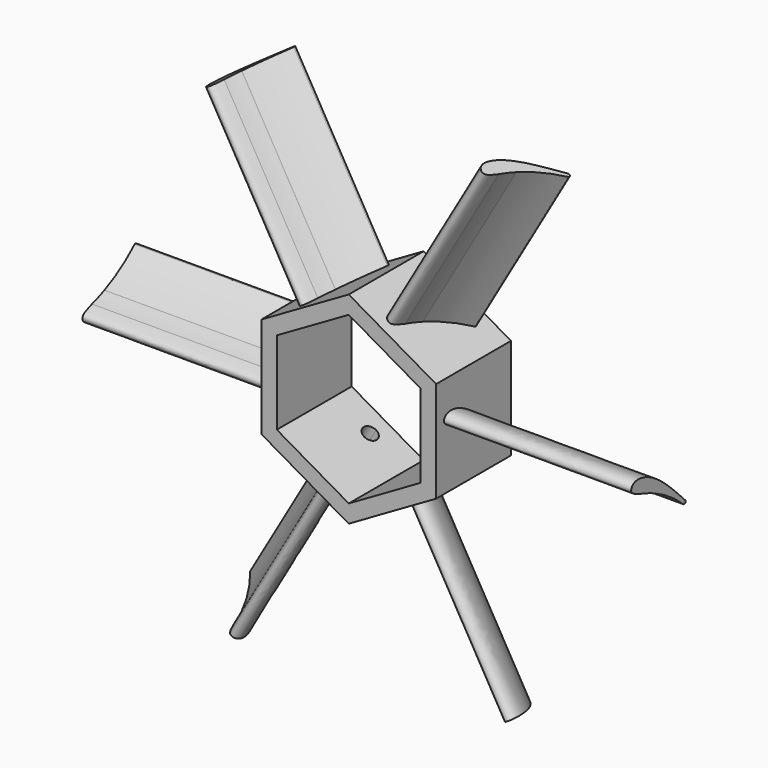
from build123d import *

# Parameters (mm, degrees)
F1_DEPTH  = 19.05
F8_DEPTH  = 38.1
F9_DEPTH  = 38.1
F10_DEPTH = 38.1
F11_DEPTH = 38.1
F12_DEPTH = 38.1
F13_DEPTH = 38.1
F15_DEPTH = 19.0510001
F16_DEPTH = 89.8612751667


# Not quite as in the source:
# - a feature of the source that left no trace in its solid (it failed there, or was rolled back) is left out


with BuildPart() as f1:
    # F0 (on Front) → F1 (new body)
    with BuildSketch(Plane.XZ):
        Polygon((17.78, -10.2652877862), (17.78, 10.2652877862), (0, 20.5305755724), (-17.78, 10.2652877862), (-17.78, -10.2652877862), (0, -20.5305755724), align=None)
    extrude(amount=F1_DEPTH)

    # F7 (on face) → F8 (join)
    with BuildSketch(Plane(origin=(-8.89, 0, 15.3979316793), x_dir=(0.8660254038, 0, 0.5), z_dir=(-0.5, 0, 0.8660254038))):
        with BuildLine():
            add(Edge.make_bspline(
                [(0, -7.7538370491), (0.0005473534, -7.7532338055), (0.0010947416, -7.7526305605), (0.0016421645, -7.7520273142)],
                knots=[0.7876107373, 0.7876107373, 0.7876107373, 0.7876107373, 0.7876968979, 0.7876968979, 0.7876968979, 0.7876968979], degree=3))
            Line((0, -7.7538370491), (0, -11.3412338568))
            ThreePointArc((0, -11.3412338568), (0.0008210147, -11.3393859842), (0.0016421645, -11.3375381715))
            Line((0.0016421645, -11.3375381715), (0.0016421645, -7.7520273142))
        make_face()
        with BuildLine():
            Line((0, -11.3412338568), (0, -7.7538370491))
            add(Edge.make_bspline(
                [(-1.1862251705, -14.5249951817), (-1.5749463751, -15.6161587285), (-2.2464066272, -17.5009876017), (-4.5376219484, -16.1747046), (-3.6264374582, -12.1661122368), (-1.1945785451, -9.0703938169), (0, -7.7538370491)],
                knots=[0, 0, 0, 0, 0.1986769511, 0.3431860009, 0.5995685898, 0.7876107373, 0.7876107373, 0.7876107373, 0.7876107373], degree=3))
            ThreePointArc((-1.1862251705, -14.5249951817), (-0.6420119978, -12.9148952786), (0, -11.3412338568))
        make_face()
        with BuildLine():
            add(Edge.make_bspline(
                [(0.0016421645, -7.7520273142), (1.3505150143, -6.2656031483), (2.9104228785, -4.7706214018), (4.4703307428, -3.2756396553)],
                knots=[0.7876968979, 0.7876968979, 0.7876968979, 0.7876968979, 1, 1, 1, 1], degree=3))
            Line((0.0016421645, -7.7520273142), (0.0016421645, -11.3375381715))
            ThreePointArc((0.0016421645, -11.3375381715), (2.2311378018, -7.2759469782), (5.1069300621, -3.6431804437))
            ThreePointArc((5.1069300621, -3.6431804437), (4.9724007966, -3.1411103898), (4.4703307428, -3.2756396553))
        make_face()
    extrude(amount=F8_DEPTH)

    # F2 (on face) → F9 (join)
    with BuildSketch(Plane(origin=(8.89, 0, 15.3979316793), x_dir=(0.8660254038, 0, -0.5), z_dir=(0.5, 0, 0.8660254038))):
        with BuildLine():
            Line((0, -11.3170660089), (0, -7.7315551515))
            add(Edge.make_bspline(
                [(-1.187867335, -14.5045230191), (-1.5765885396, -15.5956865658), (-2.2480487917, -17.4805154391), (-4.5392641129, -16.1542324374), (-3.6279463171, -12.1450536205), (-1.1952777162, -9.0487213191), (0, -7.7315551515)],
                knots=[0, 0, 0, 0, 0.1986769511, 0.3431860009, 0.5995685898, 0.7876968979, 0.7876968979, 0.7876968979, 0.7876968979], degree=3))
            ThreePointArc((-1.187867335, -14.5045230191), (-0.6429481144, -12.8925283349), (0, -11.3170660089))
        make_face()
        with BuildLine():
            add(Edge.make_bspline(
                [(0, -7.7315551515), (1.3488728498, -6.2451309857), (2.9087807141, -4.7501492392), (4.4686885783, -3.2551674926)],
                knots=[0.7876968979, 0.7876968979, 0.7876968979, 0.7876968979, 1, 1, 1, 1], degree=3))
            Line((0, -7.7315551515), (0, -11.3170660089))
            ThreePointArc((0, -11.3170660089), (2.2294956373, -7.2554748155), (5.1052878976, -3.622708281))
            ThreePointArc((5.1052878976, -3.622708281), (4.9707586321, -3.1206382272), (4.4686885783, -3.2551674926))
        make_face()
    extrude(amount=F9_DEPTH)

    # F3 (on face) → F10 (join)
    with BuildSketch(Plane.YZ.offset(17.78)):
        with BuildLine():
            add(Edge.make_bspline(
                [(-7.8599847579, 0), (-6.3747627763, -1.3481141297), (-4.8810042018, -2.9067457003), (-3.3872456274, -4.4653772708)],
                knots=[0.7878706011, 0.7878706011, 0.7878706011, 0.7878706011, 1, 1, 1, 1], degree=3))
            Line((-7.8599847579, 0), (-11.4416964799, 0))
            ThreePointArc((-11.4416964799, 0), (-7.3841573188, -2.2284377273), (-3.7547864157, -5.1019765901))
            ThreePointArc((-3.7547864157, -5.1019765901), (-3.2527163619, -4.9674473247), (-3.3872456274, -4.4653772708))
        make_face()
        with BuildLine():
            Line((-11.4416964799, 0), (-7.8599847579, 0))
            add(Edge.make_bspline(
                [(-7.8633458805, 0.0030504953), (-7.8622255112, 0.0020337834), (-7.8611051369, 0.0010169516), (-7.8599847579, 0)],
                knots=[0.7877105811, 0.7877105811, 0.7877105811, 0.7877105811, 0.7878706011, 0.7878706011, 0.7878706011, 0.7878706011], degree=3))
            Line((-7.8633458805, 0.0030504953), (-11.4485573206, 0.0030504953))
            ThreePointArc((-11.4485573206, 0.0030504953), (-11.4451267968, 0.0015254803), (-11.4416964799, 0))
        make_face()
        with BuildLine():
            Line((-11.4485573206, 0.0030504953), (-7.8633458805, 0.0030504953))
            add(Edge.make_bspline(
                [(-14.6366011538, 1.1911786424), (-15.7277647005, 1.5798998471), (-17.6125935738, 2.2513600991), (-16.2863105721, 4.5425754204), (-12.2770386202, 3.6312364543), (-9.1806088275, 1.1984392543), (-7.8633458805, 0.0030504953)],
                knots=[0, 0, 0, 0, 0.1986769511, 0.3431860009, 0.5995685898, 0.7877105811, 0.7877105811, 0.7877105811, 0.7877105811], degree=3))
            ThreePointArc((-14.6366011538, 1.1911786424), (-13.0243055984, 0.6461472944), (-11.4485573206, 0.0030504953))
        make_face()
    extrude(amount=F10_DEPTH)

    # F4 (on face) → F11 (join)
    with BuildSketch(Plane(origin=(8.89, 0, -15.3979316793), x_dir=(0.8660254038, 0, 0.5), z_dir=(0.5, 0, -0.8660254038))):
        with BuildLine():
            add(Edge.make_bspline(
                [(0, 7.7183126767), (-1.3479724171, 6.2333150924), (-2.9063657613, 4.7397848289), (-4.4647591055, 3.2462545654)],
                knots=[0.7879030237, 0.7879030237, 0.7879030237, 0.7879030237, 1, 1, 1, 1], degree=3))
            Line((0, 7.7183126767), (0, 11.2993157186))
            ThreePointArc((0, 11.2993157186), (-2.2282401234, 7.2425326354), (-5.1013584248, 3.6137953538))
            ThreePointArc((-5.1013584248, 3.6137953538), (-4.9668291593, 3.1117253), (-4.4647591055, 3.2462545654))
        make_face()
        with BuildLine():
            Line((0, 11.2993157186), (0, 7.7183126767))
            add(Edge.make_bspline(
                [(0.0039294728, 7.7226422243), (0.0026198474, 7.7211990498), (0.0013100231, 7.7197558673), (0, 7.7183126767)],
                knots=[0.7876968979, 0.7876968979, 0.7876968979, 0.7876968979, 0.7879030237, 0.7879030237, 0.7879030237, 0.7879030237], degree=3))
            Line((0.0039294728, 7.7226422243), (0.0039294728, 11.3081530816))
            ThreePointArc((0.0039294728, 11.3081530816), (0.0019651224, 11.3037342285), (0, 11.2993157186))
        make_face()
        with BuildLine():
            Line((0.0039294728, 11.3081530816), (0.0039294728, 7.7226422243))
            add(Edge.make_bspline(
                [(1.1917968078, 14.4956100919), (1.5805180124, 15.5867736386), (2.2519782645, 17.4716025119), (4.5431935857, 16.1453195102), (3.63187579, 12.1361406932), (1.199207189, 9.0398083919), (0.0039294728, 7.7226422243)],
                knots=[0, 0, 0, 0, 0.1986769511, 0.3431860009, 0.5995685898, 0.7876968979, 0.7876968979, 0.7876968979, 0.7876968979], degree=3))
            ThreePointArc((1.1917968078, 14.4956100919), (0.6468775872, 12.8836154077), (0.0039294728, 11.3081530816))
        make_face()
    extrude(amount=F11_DEPTH)

    # F5 (on face) → F12 (join)
    with BuildSketch(Plane(origin=(-8.89, 0, -15.3979316793), x_dir=(0.8660254038, 0, -0.5), z_dir=(-0.5, 0, -0.8660254038))):
        with BuildLine():
            add(Edge.make_bspline(
                [(0, 7.7773641781), (-0.0019872196, 7.7751733378), (-0.0039748984, 7.7729824789), (-0.0059630356, 7.7707916014)],
                knots=[0.787383979, 0.787383979, 0.787383979, 0.787383979, 0.7876968979, 0.7876968979, 0.7876968979, 0.7876968979], degree=3))
            Line((0, 7.7773641781), (0, 11.3697292081))
            ThreePointArc((0, 11.3697292081), (-0.0029806269, 11.3630154378), (-0.0059630356, 11.3563024588))
            Line((-0.0059630356, 11.3563024588), (-0.0059630356, 7.7707916014))
        make_face()
        with BuildLine():
            Line((0, 11.3697292081), (0, 7.7773641781))
            add(Edge.make_bspline(
                [(1.1819042994, 14.543759469), (1.570625504, 15.6349230157), (2.2420857561, 17.519751889), (4.5333010773, 16.1934688873), (3.6224674222, 12.18641996), (1.1927388288, 9.092317135), (0, 7.7773641781)],
                knots=[0, 0, 0, 0, 0.1986769511, 0.3431860009, 0.5995685898, 0.787383979, 0.787383979, 0.787383979, 0.787383979], degree=3))
            ThreePointArc((1.1819042994, 14.543759469), (0.6395493316, 12.9386483491), (0, 11.3697292081))
        make_face()
        with BuildLine():
            add(Edge.make_bspline(
                [(-0.0059630356, 7.7707916014), (-1.3548358854, 6.2843674356), (-2.9147437496, 4.7893856891), (-4.4746516139, 3.2944039425)],
                knots=[0.7876968979, 0.7876968979, 0.7876968979, 0.7876968979, 1, 1, 1, 1], degree=3))
            Line((-0.0059630356, 7.7707916014), (-0.0059630356, 11.3563024588))
            ThreePointArc((-0.0059630356, 11.3563024588), (-2.2354586728, 7.2947112654), (-5.1112509332, 3.6619447309))
            ThreePointArc((-5.1112509332, 3.6619447309), (-4.9767216677, 3.1598746771), (-4.4746516139, 3.2944039425))
        make_face()
    extrude(amount=F12_DEPTH)

    # F6 (on face) → F13 (join)
    with BuildSketch(Plane(origin=(-17.78, 0, 0), x_dir=(0, -1, 0), z_dir=(-1, 0, 0))):
        with BuildLine():
            add(Edge.make_bspline(
                [(7.7609154689, 0), (7.760325141, 0.0005356357), (7.7597348118, 0.0010713047), (7.7591444813, 0.0016070071)],
                knots=[0.7876125821, 0.7876125821, 0.7876125821, 0.7876125821, 0.7876968979, 0.7876968979, 0.7876968979, 0.7876968979], degree=3))
            Line((7.7609154689, 0), (11.348271887, 0))
            ThreePointArc((11.348271887, 0), (11.3464635841, 0.0008034389), (11.3446553386, 0.0016070071))
            Line((11.3446553386, 0.0016070071), (7.7591444813, 0.0016070071))
        make_face()
        with BuildLine():
            Line((11.348271887, 0), (7.7609154689, 0))
            add(Edge.make_bspline(
                [(14.5321123488, -1.1862603279), (15.6232758956, -1.5749815326), (17.5081047688, -2.2464417846), (16.1818217672, -4.5376571059), (12.1732168477, -3.6264697615), (9.0774852842, -1.1945935139), (7.7609154689, 0)],
                knots=[0, 0, 0, 0, 0.1986769511, 0.3431860009, 0.5995685898, 0.7876125821, 0.7876125821, 0.7876125821, 0.7876125821], degree=3))
            ThreePointArc((14.5321123488, -1.1862603279), (12.9219718729, -0.6420320383), (11.348271887, 0))
        make_face()
        with BuildLine():
            add(Edge.make_bspline(
                [(7.7591444813, 0.0016070071), (6.2727203155, 1.3504798569), (4.7777385689, 2.9103877211), (3.2827568224, 4.4702955854)],
                knots=[0.7876968979, 0.7876968979, 0.7876968979, 0.7876968979, 1, 1, 1, 1], degree=3))
            Line((7.7591444813, 0.0016070071), (11.3446553386, 0.0016070071))
            ThreePointArc((11.3446553386, 0.0016070071), (7.2830641453, 2.2311026443), (3.6502976108, 5.1068949047))
            ThreePointArc((3.6502976108, 5.1068949047), (3.148227557, 4.9723656392), (3.2827568224, 4.4702955854))
        make_face()
    extrude(amount=F13_DEPTH)

    # F14 (on face) → F15 (cut, through all)
    with BuildSketch(Plane(origin=(0, 0, 0), x_dir=(-1, 0, 0), z_dir=(0, 1, 0))):
        Polygon((-14.63675, -8.4505315526), (0, -16.9010631051), (14.63675, -8.4505315526), (14.63675, 8.4505315526), (0, 16.9010631051), (-14.63675, 8.4505315526), align=None)
    extrude(amount=-F15_DEPTH, mode=Mode.SUBTRACT)

    # F2 (on face) → F16 (cut, through all)
    with BuildSketch(Plane(origin=(8.89, 0, 15.3979316793), x_dir=(0.8660254038, 0, -0.5), z_dir=(0.5, 0, 0.8660254038))):
        with BuildLine():
            ThreePointArc((1.5, -4.445), (1.0606601718, -3.3843398282), (0, -2.945))
            Line((0, -2.945), (0, -4.445))
            Line((0, -4.445), (0, -5.945))
            ThreePointArc((0, -5.945), (1.0606601718, -5.5056601718), (1.5, -4.445))
        make_face()
        with BuildLine():
            Line((0, -4.445), (0, -2.945))
            ThreePointArc((0, -2.945), (-1.5, -4.445), (0, -5.945))
            Line((0, -5.945), (0, -4.445))
        make_face()
    extrude(amount=-F16_DEPTH, mode=Mode.SUBTRACT)


solid = f1.part
